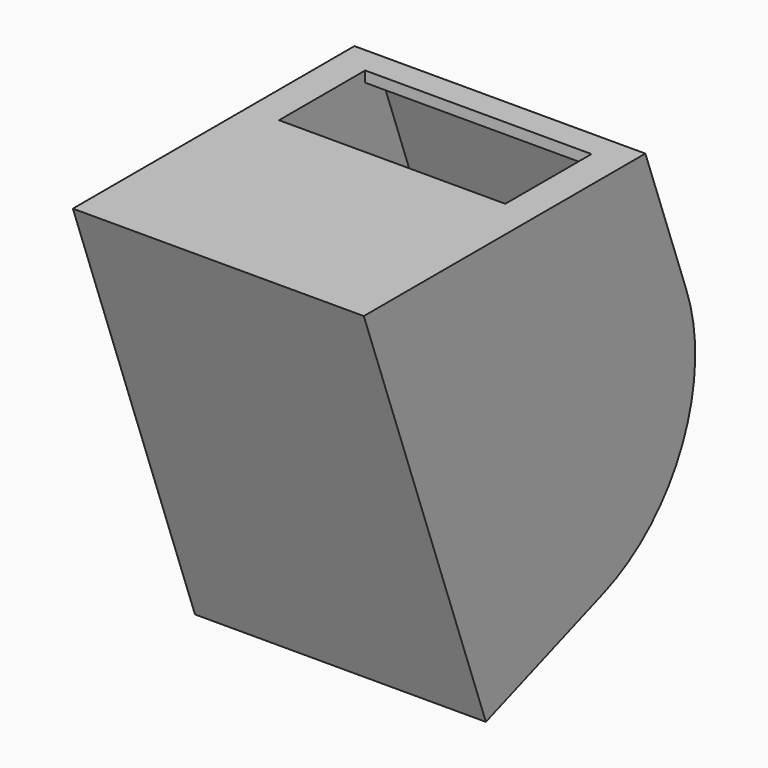
from build123d import *

# Parameters (mm, degrees)
F0_W      = 53.34
F0_H      = 25.4
F0_R      = 1.27
F1_DEPTH  = 2.54
F3_DEPTH  = 53.34
F5_DEPTH  = 7.62
F6_W      = 12.7
F6_H      = 8.89
F7_DEPTH  = 7.62
F8_W      = 12.7
F8_H      = 2.54
F9_DEPTH  = 9.525
F10_W     = 68.58
F10_H     = 41.6090539173
F11_DEPTH = 2.54
F13_REACH = 169.3857709485
F15_DEPTH = 63.5
F17_DEPTH = 2.54
F19_DEPTH = 2.54
F21_DEPTH = 2.54
F22_W     = 63.5
F22_H     = 2.54


with BuildPart() as f1:
    # F0 (on Top) → F1 (new body)
    with BuildSketch(Plane.XY):
        Rectangle(F0_W, F0_H)
        with Locations((-22.86, -8.89)):
            Circle(F0_R, mode=Mode.SUBTRACT)
        with Locations((22.86, -8.89)):
            Circle(F0_R, mode=Mode.SUBTRACT)
        with Locations((-22.86, 8.89)):
            Circle(F0_R, mode=Mode.SUBTRACT)
        with Locations((22.86, 8.89)):
            Circle(F0_R, mode=Mode.SUBTRACT)
    extrude(amount=F1_DEPTH)

    # F2 (on face) → F3 (join, through all)
    with BuildSketch(Plane.YZ.offset(26.67)):
        Polygon((-15.24, -0.447870531), (-9.9437557743, -14.9991819491), (-7.5569365175, -14.130450785), (-12.7, 0), (-12.7, 2.54), (-12.7, 33.02), (-27.4213086776, 33.02), (-26.4968242825, 30.48), (-15.24, 30.48), align=None)
        Polygon((-26.4968242825, 30.48), (-15.24, -0.447870531), (-15.24, 30.48), align=None)
    extrude(amount=-F3_DEPTH)



with BuildPart() as f3:
    # F2 (on face) → F3, piece 2 (new body, through all)
    with BuildSketch(Plane.YZ.offset(26.67)):
        Polygon((12.7, 33.02), (12.7, 30.48), (17.2714728529, 30.48), (28.7046231961, -0.9323224012), (31.0914424529, -0.0635912371), (19.05, 33.02), align=None)
    extrude(amount=-F3_DEPTH)


with BuildPart() as f1_1:
    add(f1.part)

    add(f3.part)  # F5 merges F3
    # F4 (on face) → F5 (join)
    with BuildSketch(Plane.YZ.offset(26.67)):
        Polygon((-27.4213086776, 33.02), (-9.9437557743, -14.9991819491), (31.0914424529, -0.0635912371), (19.05, 33.02), align=None)
    extrude(amount=F5_DEPTH)

    # F6 (on face) → F7 (join)
    with BuildSketch(Plane(origin=(-26.67, 0, 0), x_dir=(0, -1, 0), z_dir=(-1, 0, 0))):
        Polygon((9.9437557743, -14.9991819491), (27.4213086776, 33.02), (-19.05, 33.02), (-31.0914424529, -0.0635912371), align=None)
        with Locations((0, 6.985)):
            Rectangle(F6_W, F6_H, mode=Mode.SUBTRACT)
    extrude(amount=F7_DEPTH)

    # F8 (on face) → F9 (cut)
    with BuildSketch(Plane(origin=(-34.29, 0, 0), x_dir=(0, -1, 0), z_dir=(-1, 0, 0))):
        with Locations((0, 1.27)):
            Rectangle(F8_W, F8_H)
    extrude(amount=-F9_DEPTH, mode=Mode.SUBTRACT)

    # F10 (on face) → F11 (join, through all)
    with BuildSketch(Plane(origin=(0, -13.6012014706, -4.9504324856), x_dir=(1, 0, 0), z_dir=(0, -0.9396926208, -0.3420201433))):
        with Locations((0, -31.4981827789)):
            Rectangle(F10_W, F10_H)
    extrude(amount=-F11_DEPTH)

    f13_end = Plane(origin=(0, -7.2808291762, 33.02), x_dir=(1, 0, 0), z_dir=(0, 0, 1))
    # F12 (on face) → F13 (join, up to a plane its end follows)
    with BuildSketch(Plane(origin=(0, 17.8885802808, -49.1484703875), x_dir=(1, 0, 0), z_dir=(0, 0.3420201433, -0.9396926208))):
        Polygon((31.75, 14.474096284), (34.29, 14.474096284), (34.29, 48.764096284), (-34.29, 48.764096284), (-34.29, 14.474096284), (-31.75, 14.474096284), (-31.75, 46.224096284), (31.75, 46.224096284), align=None)
    f13_long = extrude(amount=-F13_REACH, mode=Mode.PRIVATE)
    add(split(f13_long, bisect_by=f13_end, keep=Keep.BOTTOM, mode=Mode.PRIVATE))

    # F14 (on face) → F15 (join, through all)
    with BuildSketch(Plane(origin=(31.75, 0, 0), x_dir=(0, -1, 0), z_dir=(-1, 0, 0))):
        Polygon((27.4213086775, 33.02), (26.5525775135, 30.6331807432), (60.3402217897, 30.6331807432), (61.2089529537, 33.02), align=None)
    extrude(amount=F15_DEPTH)

    # F16 (on face) → F17 (cut, through all)
    with BuildSketch(Plane(origin=(0, -11.2143822138, -4.0817013215), x_dir=(-1, 0, 0), z_dir=(0, 0.9396926208, 0.3420201433))):
        Polygon((26.67, 4.3436558202), (-26.67, 4.3436558202), (-26.67, -10.6936558203), (-31.75, -10.6936558203), (-31.75, -52.3027097376), (31.75, -52.3027097376), (31.75, -10.6936558203), (26.67, -10.6936558203), align=None)
    extrude(amount=-F17_DEPTH, mode=Mode.SUBTRACT)

    # F18 (on face) → F19 (join)
    with BuildSketch(Plane.YZ.offset(34.29)):
        with BuildLine():
            ThreePointArc((6.6741980668, -53.230171709), (29.9844867323, -31.7454245982), (31.0914424529, -0.0635912371))
            Line((31.0914424529, -0.0635912371), (-7.5569365175, -14.130450785))
            Line((-7.5569365176, -14.130450785), (6.6741980668, -53.230171709))
        make_face()
    extrude(amount=-F19_DEPTH)

    # F20 (on face) → F21 (join)
    with BuildSketch(Plane(origin=(-34.29, 0, 0), x_dir=(0, -1, 0), z_dir=(-1, 0, 0))):
        with BuildLine():
            ThreePointArc((-31.0914424529, -0.0635912371), (-29.9844867323, -31.7454245982), (-6.6741980668, -53.230171709))
            Line((-6.6741980669, -53.230171709), (7.5569365175, -14.130450785))
            Line((7.5569365175, -14.130450785), (-31.0914424529, -0.0635912371))
        make_face()
    extrude(amount=-F21_DEPTH)

    # F24: sweep along a path in F23
    with BuildLine(Plane(origin=(31.75, 0, 0), x_dir=(0, -1, 0), z_dir=(-1, 0, 0))) as f24_path:
        ThreePointArc((-18.5834505022, -46.4695330224), (-32.3206049052, -25.2835298235), (-31.0914424529, -0.0635912371))
    # F22 (on face) → F24 (sweep)
    with BuildSketch(Plane(origin=(0, 3.6574456963, -10.0487494635), x_dir=(1, 0, 0), z_dir=(0, 0.3420201433, -0.9396926208))):
        with Locations((0, -27.9246495586)):
            Rectangle(F22_W, F22_H)
    sweep(path=f24_path.line)


solid = f1_1.part
